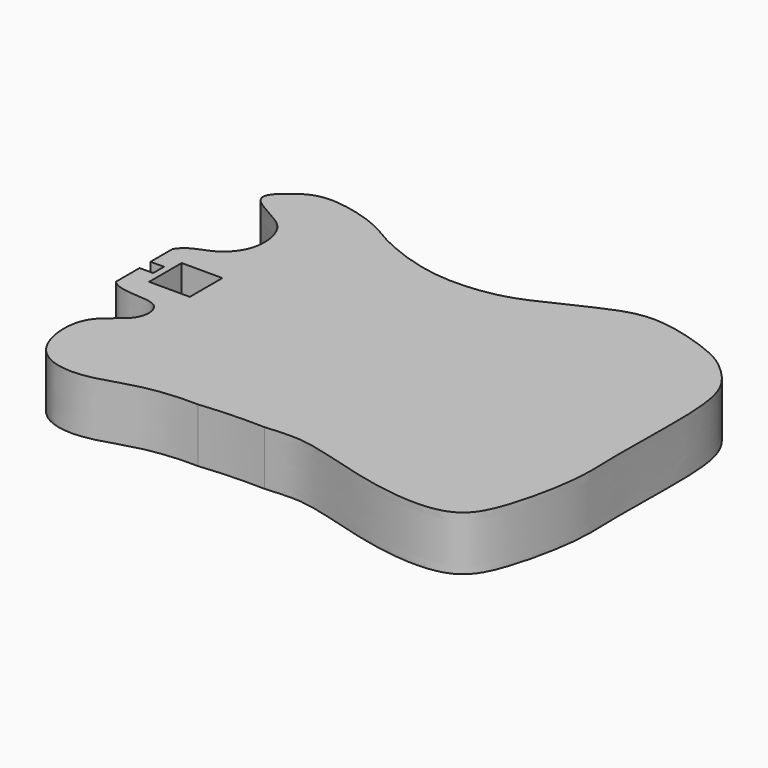
from build123d import *

# Parameters (mm, degrees)
F0_W     = 38.1
F0_H     = 38.1
F1_DEPTH = 50.8


with BuildPart() as f1:
    # F0 (on Top) → F1 (new body)
    with BuildSketch(Plane.XY):
        with BuildLine():
            Line((-228.6, 32.1917161345), (-228.6, 6.35))
            Line((-228.6, 6.35), (-215.9, 6.35))
            Line((-215.9, 6.35), (-215.9, -6.35))
            Line((-215.9, -6.35), (-228.6, -6.35))
            Line((-228.6, -6.35), (-228.6, -34.1989696026))
            add(Edge.make_bspline(
                [(-60.5002641678, -148.1617689133), (-66.5005939975, -148.1920038294), (-73.2961742589, -147.7400798137), (-113.8053654337, -150.7602742609), (-159.0025882902, -170.6546271451), (-210.2629173909, -157.2359768705), (-217.554857804, -88.5993198257), (-176.493256404, -74.2755969971), (-178.6218818379, -34.4669105888), (-217.486655562, -44.8664744461), (-228.6, -34.1989696026)],
                knots=[0.7551474079, 0.7551474079, 0.7551474079, 0.7551474079, 0.7709603375, 0.797321274, 0.8281985508, 0.8569640319, 0.8887766406, 0.9150101165, 0.9359092043, 0.9648400573, 0.9648400573, 0.9648400573, 0.9648400573], degree=3))
            ThreePointArc((-60.5002641678, -148.1617689133), (-30.426607809, -146.014377891), (-0.2766438162, -145.8888142753))
            add(Edge.make_bspline(
                [(-228.6, 32.1917161345), (-221.842404284, 42.7562656596), (-202.2675149277, 44.3254987929), (-179.2330180071, 69.4717636205), (-185.0075932705, 107.0495276869), (-206.3151011845, 119.2412421658), (-237.2938577645, 135.5477688838), (-214.5215066994, 156.5638416404), (-191.1558469206, 170.1168033125), (-137.9504249958, 156.2201135467), (-117.4820801505, 140.5399957432), (-69.4089325992, 121.1981346936), (-26.1295527608, 118.3192775912), (13.3922603976, 125.0054796597), (44.1790163062, 140.8740829992), (75.3340703353, 155.1567259182), (114.979025581, 172.0791756849), (180.9319317383, 150.3972339265), (198.7233235329, 137.7992502734), (222.9592193706, 114.3998560963), (231.0968349346, 69.5357158437), (227.151302935, -14.8262371264), (231.4981557673, -63.3730305184), (217.6910113022, -130.9001658988), (195.5401577855, -175.3182842089), (113.225990128, -168.7347991647), (39.6261978432, -141.9301941848), (15.666877208, -144.8577880121), (-0.1842328972, -145.8828575521), (-0.2766438162, -145.8888142753)],
                knots=[0, 0, 0, 0, 0.023526495, 0.0472150591, 0.071976495, 0.0937567881, 0.1160251968, 0.1361214471, 0.1589295174, 0.1896491945, 0.2123633437, 0.2426795653, 0.2715030285, 0.2984604786, 0.3236752725, 0.3486429477, 0.3768921666, 0.4118773119, 0.4324349076, 0.4559076572, 0.4849876683, 0.5244190328, 0.5554779008, 0.5907664036, 0.6188059718, 0.6563222449, 0.6944312953, 0.721571422, 0.7217302364, 0.7217302364, 0.7217302364, 0.7217302364], degree=3))
        make_face()
        with Locations((-190.5, 0)):
            Rectangle(F0_W, F0_H, mode=Mode.SUBTRACT)
    extrude(amount=F1_DEPTH)


solid = f1.part
